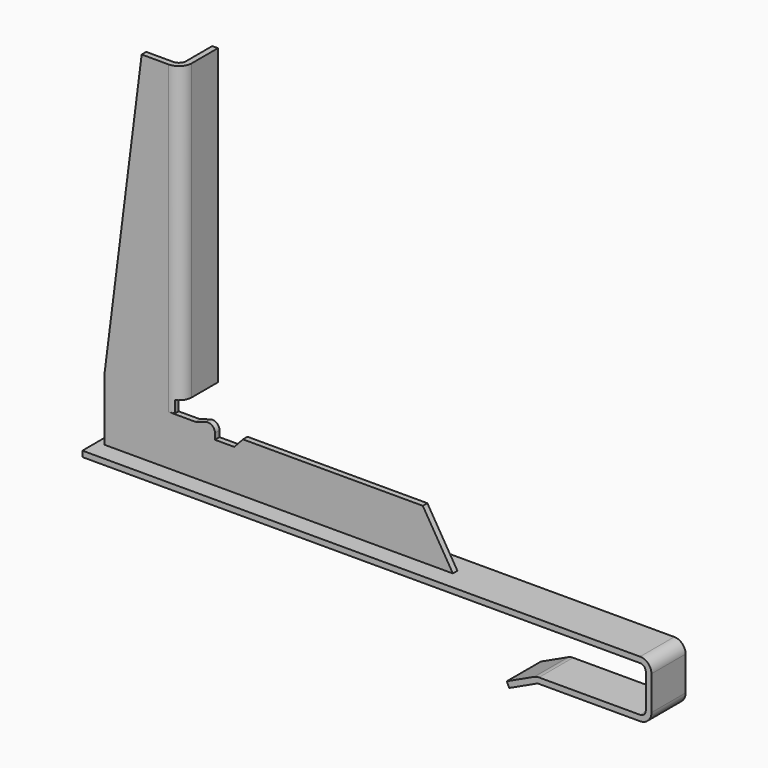
from build123d import *

# Parameters (mm, degrees)
F1_DEPTH    = 15
F3_DEPTH    = 2
F4_W        = 4
F4_H        = 28
F5_DEPTH    = 206.7509774754
F6_T1_DEPTH = 206.7509774754
F7_T4_DEPTH = 251.7509774754


# Not quite as in the source:
# - a fillet or chamfer that OpenCascade refuses, or shapes differently, is made with other operations: its cross-section is extruded or revolved along the edge and cut away or added


with BuildPart() as f1:
    # F0 (on Front) → F1 (new body, symmetric)
    with BuildSketch(Plane.XZ):
        with BuildLine():
            Line((180.6789295077, 32.8460444401), (-211.3210704923, 32.8460444401))
            Line((-211.3210704923, 32.8460444401), (-211.3210704923, 28.8460444401))
            Line((-211.3210704923, 28.8460444401), (180.6789295077, 28.8460444401))
            ThreePointArc((180.6789295077, 28.8460444401), (183.5073566325, 27.6744715648), (184.6789295077, 24.8460444401))
            Line((184.6789295077, 24.8460444401), (184.6789295077, 0.8460444401))
            ThreePointArc((184.6789295077, 0.8460444401), (183.5073566325, -1.9823826847), (180.6789295077, -3.1539555599))
            Line((180.6789295077, -3.1539555599), (109.5657081583, -3.1539555599))
            ThreePointArc((109.5657081583, -3.1539555599), (107.8341912468, -3.343587503), (106.1847620644, -3.9034932637))
            Line((106.1847620644, -3.9034932637), (86.9884564608, -12.8548775749))
            Line((86.9884564608, -12.8548775749), (88.6789295077, -16.480108723))
            Line((88.6789295077, -16.480108723), (107.8752351113, -7.5287244118))
            ThreePointArc((107.8752351113, -7.5287244118), (108.6999497026, -7.2487715315), (109.5657081583, -7.1539555599))
            Line((109.5657081583, -7.1539555599), (180.6789295077, -7.1539555599))
            ThreePointArc((180.6789295077, -7.1539555599), (186.3357837572, -4.8108098094), (188.6789295077, 0.8460444401))
            Line((188.6789295077, 0.8460444401), (188.6789295077, 24.8460444401))
            ThreePointArc((188.6789295077, 24.8460444401), (186.3357837572, 30.5028986895), (180.6789295077, 32.8460444401))
        make_face()
    extrude(amount=F1_DEPTH, both=True)

    # F2 (on Front) → F3 (join, symmetric)
    with BuildSketch(Plane.XZ):
        with BuildLine():
            Line((-206.3210704923, 75.6694748998), (-206.3210704923, 32.8460444401))
            Line((-206.3210704923, 32.8460444401), (38.6789295077, 32.8460444401))
            Line((38.6789295077, 32.8460444401), (17.569155556, 67.8460444401))
            Line((17.569155556, 67.8460444401), (-108.8612323146, 67.8460444401))
            Line((-108.8612323146, 67.8460444401), (-115.0114574584, 61.1853342652))
            Line((-115.0114574584, 61.1853342652), (-128.5433099752, 61.1853342652))
            Line((-128.5433099752, 61.1853342652), (-128.5433099752, 65.3464212941))
            ThreePointArc((-128.5433099752, 65.3464212941), (-130.579832864, 69.3735546928), (-135.0304313397, 70.1201483545))
            Line((-135.0304313397, 70.1201483545), (-142.3304080963, 67.8460444401))
            Line((-142.3304080963, 67.8460444401), (-157.2653103035, 67.8460444401))
            Line((-157.2653103035, 67.8460444401), (-157.2653103035, 76.0950669646))
            Line((-157.2653103035, 76.0950669646), (-152.0575187367, 76.0950669646))
            Line((-152.0575187367, 76.0950669646), (-152.0575187367, 282.8460444401))
            Line((-152.0575187367, 282.8460444401), (-180.0575187367, 282.8460444401))
            Line((-180.0575187367, 282.8460444401), (-206.3210704923, 75.6694748998))
        make_face()
    extrude(amount=F3_DEPTH, both=True)

    # F4 (on face) → F5 (join, through all)
    with BuildSketch(Plane.XY.offset(282.8460444401)):
        with Locations((-154.0575187367, 16)):
            Rectangle(F4_W, F4_H)
    extrude(amount=-F5_DEPTH)

    # F6: fillet of radius 5 on 1 edges, made by hand

    # F6_s2 → F6_t1 (join)
    with BuildSketch(Plane.XY.offset(76.0950669646)):
        with BuildLine():
            ThreePointArc((-161.0575187367, 2), (-157.5219848308, 3.4644660941), (-156.0575187367, 7))
            Line((-156.0575187367, 7), (-156.0575187367, 2))
            Line((-156.0575187367, 2), (-161.0575187367, 2))
        make_face()
    extrude(amount=F6_T1_DEPTH)

    # F7: fillet of radius 9 on 1 edges, made by hand


with BuildPart() as f7_tool2:
    # F7_s3 → F7_t4 (new body)
    with BuildSketch(Plane.XY.offset(53.5950669646)):
        with BuildLine():
            ThreePointArc((-161.0575187367, -2), (-154.6935577061, 0.6360389693), (-152.0575187367, 7))
            Line((-152.0575187367, 7), (-152.0575187367, -2))
            Line((-152.0575187367, -2), (-161.0575187367, -2))
        make_face()
    extrude(amount=F7_T4_DEPTH)

    split(bisect_by=Plane.XY.offset(67.8460444401), keep=Keep.TOP)


with BuildPart() as f1_1:
    add(f1.part)

    # F7_t1: cut F7_tool2
    add(f7_tool2.part, mode=Mode.SUBTRACT)


solid = f1_1.part
